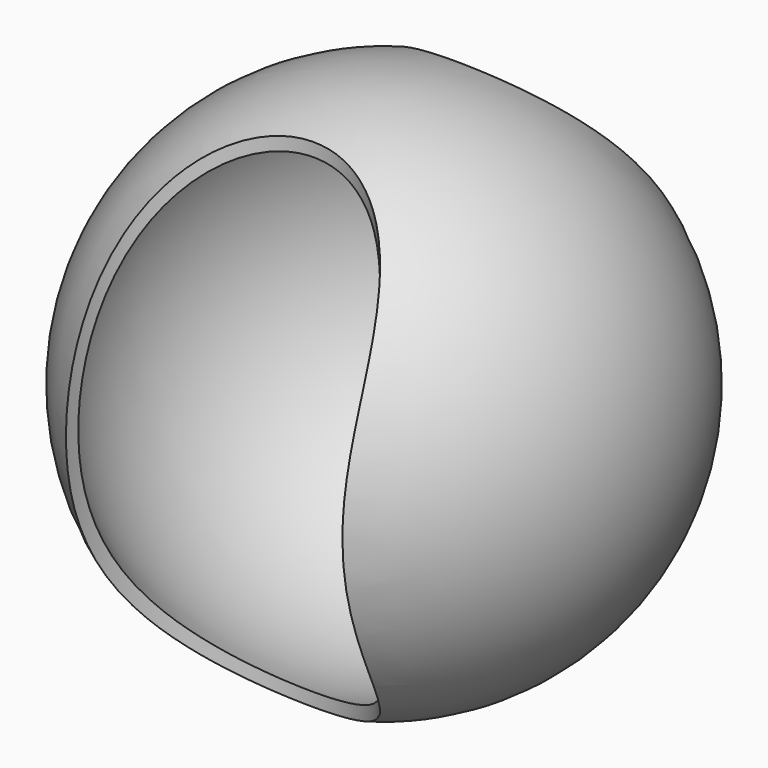
from build123d import *

# Parameters (mm, degrees)
F2_R     = 27.94
F3_DEPTH = 63.5


# Not quite as in the source:
# - the program builds the solid bodies; features that only make, move or delete a surface that nothing else refers to are left out


with BuildPart() as f1:
    # F0 (on Front) → F1 (revolve)
    with BuildSketch(Plane.XZ):
        with BuildLine():
            ThreePointArc((0, -50.8), (-50.8, 0), (0, 50.8))
            Line((0, 50.8), (0, 53.34))
            ThreePointArc((0, 53.34), (-53.34, 0), (0, -53.34))
            Line((0, -53.34), (0, -50.8))
        make_face()
    revolve(axis=Axis((0, 0, -2.3532360792), (0, 0, -1)))

    # F2 (on Top) → F3 (cut, symmetric)
    with BuildSketch(Plane.XY):
        with Locations((0, 45.72)):
            Circle(F2_R)
        with Locations((0, -45.72)):
            Circle(F2_R)
    extrude(amount=F3_DEPTH, both=True, mode=Mode.SUBTRACT)


solid = f1.part
